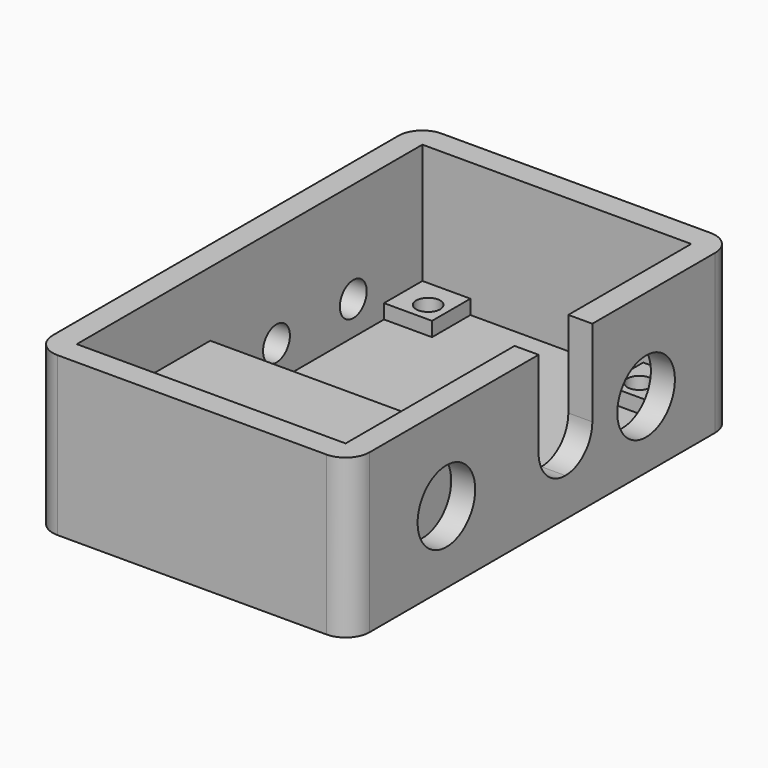
from build123d import *

# Parameters (mm, degrees)
F0_W         = 66
F0_H         = 100
F0_W_2       = 50
F0_H_2       = 26
F0_W_3       = 15
F0_H_3       = 12
F0_W_4       = 14
F0_H_4       = 10
F0_W_5       = 36
F0_H_5       = 2
F0_W_6       = 8
F0_H_6       = 8
F0_R         = 2.5
F1_DEPTH     = 5
F2_DEPTH     = 28
F3_DEPTH     = 3
F5_DEPTH     = 17
F6_R         = 5
F7_DEPTH     = 25
F8_R         = 7.5
F9_DEPTH     = 25
F10_DEPTH    = 10
F4_W         = 5
F4_H         = 14
F11_DEPTH    = 25
F12_T1_DEPTH = 5
F13_R        = 3.5
F14_DEPTH    = 25


# Not quite as in the source:
# - a fillet or chamfer that OpenCascade refuses, or shapes differently, is made with other operations: its cross-section is extruded or revolved along the edge and cut away or added


with BuildPart() as f1:
    # F0 (on Top) → F1 (new body)
    with BuildSketch(Plane.XY):
        with Locations((0, -17)):
            Rectangle(F0_W, F0_H)
        Polygon((-18, 28), (18, 28), (28, 28), (28, 18), (28, -18), (28, -28), (28, -62), (-28, -62), (-28, -28), (-28, -18), (-28, 18), (-28, 28), align=None, mode=Mode.SUBTRACT)
        Polygon((28, -62), (28, -28), (18, -28), (-18, -28), (-28, -28), (-28, -62), align=None)
        Polygon((25, -31), (25, -57), (25, -59), (-27, -59), (-27, -29), (25, -29), align=None, mode=Mode.SUBTRACT)
        Polygon((18, 18), (18, 26), (-18, 26), (-18, 18), (-26, 18), (-26, 16), (-11, 16), (-11, 4), (-26, 4), (-26, -4), (-11, -4), (-11, -16), (-26, -16), (-26, -18), (-18, -18), (-18, -26), (18, -26), (18, -18), (13, -18), (13, -4), (26, -4), (26, 5), (12, 5), (12, 15), (26, 15), (26, 18), align=None)
        Polygon((-4, 9), (1, 9), (1, 4), (1, -1), (-4, -1), (-9, -1), (-9, 4), (-9, 9), align=None, mode=Mode.SUBTRACT)
        with Locations((0, -44)):
            Rectangle(F0_W_2, F0_H_2)
        Polygon((25, -59), (25, -57), (-25, -57), (-25, -31), (25, -31), (25, -29), (-27, -29), (-27, -59), align=None)
        Polygon((26, -18), (26, -4), (13, -4), (13, -18), (18, -18), align=None)
        with Locations((-18.5, -10)):
            Rectangle(F0_W_3, F0_H_3)
        with Locations((-18.5, 10)):
            Rectangle(F0_W_3, F0_H_3)
        with Locations((19, 10)):
            Rectangle(F0_W_4, F0_H_4)
        with BuildLine():
            ThreePointArc((1, 4), (-0.4644660941, 7.5355339059), (-4, 9))
            ThreePointArc((-4, 9), (-7.5355339059, 7.5355339059), (-9, 4))
            ThreePointArc((-9, 4), (-7.5355339059, 0.4644660941), (-4, -1))
            ThreePointArc((-4, -1), (-0.4644660941, 0.4644660941), (1, 4))
        make_face()
        with Locations((0, 27)):
            Rectangle(F0_W_5, F0_H_5)
        Polygon((28, 18), (26, 18), (26, 15), (26, 5), (26, -4), (26, -18), (28, -18), align=None)
        with Locations((0, -27)):
            Rectangle(F0_W_5, F0_H_5)
        Polygon((-26, 16), (-26, 18), (-28, 18), (-28, -18), (-26, -18), (-26, -16), (-26, -4), (-26, 4), align=None)
        with Locations((-22, 22)):
            Rectangle(F0_W_6, F0_H_6)
        with Locations((-22, 22)):
            Circle(F0_R, mode=Mode.SUBTRACT)
        with Locations((22, 22)):
            Rectangle(F0_W_6, F0_H_6)
        with Locations((22, 22)):
            Circle(F0_R, mode=Mode.SUBTRACT)
        with Locations((22, -22)):
            Rectangle(F0_W_6, F0_H_6)
        with Locations((22, -22)):
            Circle(F0_R, mode=Mode.SUBTRACT)
        with Locations((-22, -22)):
            Rectangle(F0_W_6, F0_H_6)
        with Locations((-22, -22)):
            Circle(F0_R, mode=Mode.SUBTRACT)
        Polygon((-26, 26), (-18, 26), (-18, 28), (-28, 28), (-28, 18), (-26, 18), align=None)
        Polygon((18, 26), (26, 26), (26, 18), (28, 18), (28, 28), (18, 28), align=None)
        Polygon((28, -28), (28, -18), (26, -18), (26, -26), (18, -26), (18, -28), align=None)
        Polygon((-26, -18), (-28, -18), (-28, -28), (-18, -28), (-18, -26), (-26, -26), align=None)
        with Locations((-22, 22)):
            Circle(F0_R)
        with Locations((-22, -22)):
            Circle(F0_R)
        with Locations((22, 22)):
            Circle(F0_R)
        with Locations((22, -22)):
            Circle(F0_R)
        with BuildLine():
            ThreePointArc((-4, -1), (-7.5355339059, 0.4644660941), (-9, 4))
            Line((-9, 4), (-9, -1))
            Line((-9, -1), (-4, -1))
        make_face()
        with BuildLine():
            Line((1, 4), (1, 9))
            Line((1, 9), (-4, 9))
            ThreePointArc((-4, 9), (-0.4644660941, 7.5355339059), (1, 4))
        make_face()
        with BuildLine():
            ThreePointArc((-9, 4), (-7.5355339059, 7.5355339059), (-4, 9))
            Line((-4, 9), (-9, 9))
            Line((-9, 9), (-9, 4))
        make_face()
        with BuildLine():
            Line((1, -1), (1, 4))
            ThreePointArc((1, 4), (-0.4644660941, 0.4644660941), (-4, -1))
            Line((-4, -1), (1, -1))
        make_face()
    extrude(amount=-F1_DEPTH)

    # F0 (on Top) → F2 (join)
    with BuildSketch(Plane.XY):
        with Locations((0, -17)):
            Rectangle(F0_W, F0_H)
        Polygon((-18, 28), (18, 28), (28, 28), (28, 18), (28, -18), (28, -28), (28, -62), (-28, -62), (-28, -28), (-28, -18), (-28, 18), (-28, 28), align=None, mode=Mode.SUBTRACT)
    extrude(amount=F2_DEPTH)

    # F0 (on Top) → F3 (join)
    with BuildSketch(Plane.XY):
        with Locations((-22, 22)):
            Rectangle(F0_W_6, F0_H_6)
        with Locations((-22, 22)):
            Circle(F0_R, mode=Mode.SUBTRACT)
        Polygon((-26, 26), (-18, 26), (-18, 28), (-28, 28), (-28, 18), (-26, 18), align=None)
        Polygon((18, 26), (26, 26), (26, 18), (28, 18), (28, 28), (18, 28), align=None)
        with Locations((22, 22)):
            Rectangle(F0_W_6, F0_H_6)
        with Locations((22, 22)):
            Circle(F0_R, mode=Mode.SUBTRACT)
        Polygon((-26, -18), (-28, -18), (-28, -28), (-18, -28), (-18, -26), (-26, -26), align=None)
        with Locations((-22, -22)):
            Rectangle(F0_W_6, F0_H_6)
        with Locations((-22, -22)):
            Circle(F0_R, mode=Mode.SUBTRACT)
        Polygon((28, -28), (28, -18), (26, -18), (26, -26), (18, -26), (18, -28), align=None)
        with Locations((22, -22)):
            Rectangle(F0_W_6, F0_H_6)
        with Locations((22, -22)):
            Circle(F0_R, mode=Mode.SUBTRACT)
    extrude(amount=F3_DEPTH)

    # F6
    f6_edges = [f1.edges().sort_by_distance(p)[0] for p in [
        (-33, 33, 11.5),
        (-33, -67, 11.5),
        (33, -67, 11.5),
        (33, 33, 11.5),
    ]]
    fillet(f6_edges, radius=F6_R)

    # F0 (on Top) → F7 (cut)
    with BuildSketch(Plane.XY):
        with Locations((22, 22)):
            Circle(F0_R)
        with Locations((22, -22)):
            Circle(F0_R)
        with Locations((-22, -22)):
            Circle(F0_R)
        with Locations((-22, 22)):
            Circle(F0_R)
    extrude(amount=-F7_DEPTH, mode=Mode.SUBTRACT)

    # F8 (on face) → F9 (cut)
    with BuildSketch(Plane.YZ.offset(33)):
        with Locations((-42, 10)):
            Circle(F8_R)
        with Locations((10, 9)):
            Circle(F8_R)
    extrude(amount=-F9_DEPTH, mode=Mode.SUBTRACT)

    # F0 (on Top) → F10 (join)
    with BuildSketch(Plane.XY):
        Polygon((25, -59), (25, -57), (-25, -57), (-25, -31), (25, -31), (25, -29), (-27, -29), (-27, -59), align=None)
    extrude(amount=F10_DEPTH)

    # F4 (on face) → F11 (cut)
    with BuildSketch(Plane.XY.offset(28)):
        with Locations((30.5, -11)):
            Rectangle(F4_W, F4_H)
    extrude(amount=-F11_DEPTH, mode=Mode.SUBTRACT)

    # F12: fillet of radius 7 on 2 edges, made by hand

    # F12_s2 → F12_t1 (join)
    with BuildSketch(Plane.YZ.offset(28)):
        with BuildLine():
            ThreePointArc((-11, 3), (-6.0502525317, 5.0502525317), (-4, 10))
            Line((-4, 10), (-4, 3))
            Line((-4, 3), (-11, 3))
        make_face()
        with BuildLine():
            ThreePointArc((-18, 10), (-15.9497474683, 5.0502525317), (-11, 3))
            Line((-11, 3), (-18, 3))
            Line((-18, 3), (-18, 10))
        make_face()
    extrude(amount=F12_T1_DEPTH)

    # F13 (on face) → F14 (cut)
    with BuildSketch(Plane(origin=(-33, 0, 0), x_dir=(0, -1, 0), z_dir=(-1, 0, 0))):
        with Locations((-10, 7)):
            Circle(F13_R)
        with Locations((10, 7)):
            Circle(F13_R)
    extrude(amount=-F14_DEPTH, mode=Mode.SUBTRACT)


with BuildPart() as f5:
    # F0 (on Top) → F5 (new body)
    with BuildSketch(Plane.XY):
        with Locations((0, -44)):
            Rectangle(F0_W_2, F0_H_2)
    extrude(amount=F5_DEPTH)


solid = Compound([f1.part, f5.part])
